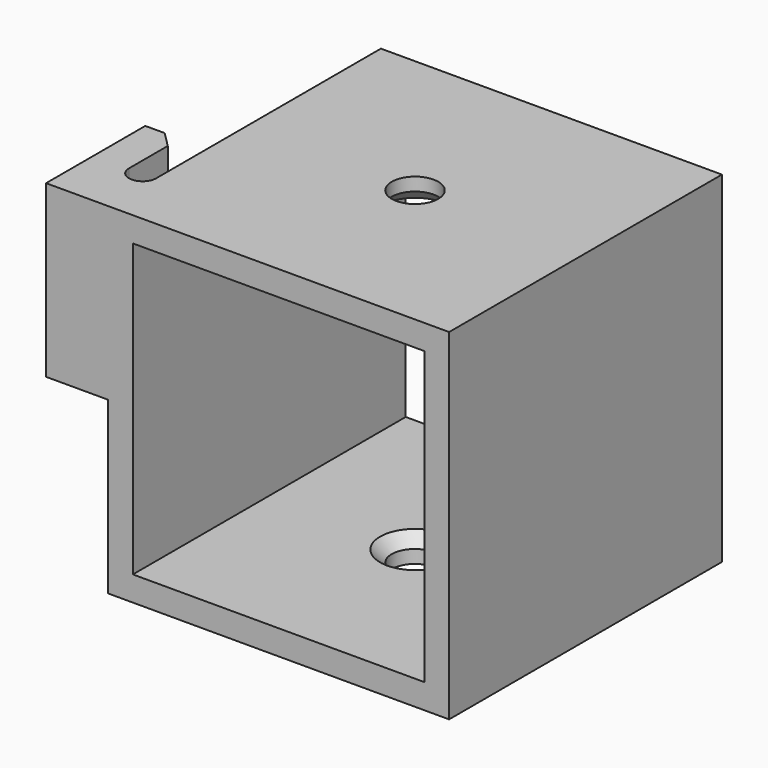
from build123d import *

# Parameters (mm, degrees)
F0_W     = 22
F0_H     = 22
F0_W_2   = 18.8
F0_H_2   = 18.8
F1_DEPTH = 11
F2_R     = 1.5
F3_DEPTH = 25
F4_SIZE  = 0.75
F6_DEPTH = 11
F7_R     = 0.87499
F8_SIZE  = 1


# Not quite as in the source:
# - a fillet or chamfer is up to 0.001 mm smaller than in the source, because OpenCascade refuses the exact size


with BuildPart() as f1:
    # F0 (on Front) → F1 (new body, symmetric)
    with BuildSketch(Plane.XZ):
        Rectangle(F0_W, F0_H)
        Rectangle(F0_W_2, F0_H_2, mode=Mode.SUBTRACT)
    extrude(amount=F1_DEPTH, both=True)

    # F2 (on face) → F3 (cut)
    with BuildSketch(Plane.XY.offset(11)):
        Circle(F2_R)
    extrude(amount=-F3_DEPTH, mode=Mode.SUBTRACT)

    # F4
    f4_edges = [f1.edges().sort_by_distance(p)[0] for p in [
        (-1.5, 0, -9.4),
        (-1.5, 0, 9.4),
    ]]
    chamfer(f4_edges, length=F4_SIZE)

    # F5 (on Top) → F6 (join, through all)
    with BuildSketch(Plane.XY):
        Polygon((-12.75, -3), (-15, -3), (-15, -11), (-11, -11), (-11, -8), (-12.75, -8), align=None)
    extrude(amount=F6_DEPTH)

    # F7 (radius 0.875 in the source; OpenCascade refuses exactly that, so slightly less here)
    f7_edges = [f1.edges().sort_by_distance(p)[0] for p in [
        (-12.75, -8, 5.5),
        (-11, -8, 5.5),
    ]]
    fillet(f7_edges, radius=F7_R)

    # F8
    f8_edges = [f1.edges().sort_by_distance(p)[0] for p in [
        (-12.75, -3, 5.5),
    ]]
    chamfer(f8_edges, length=F8_SIZE)


solid = f1.part
